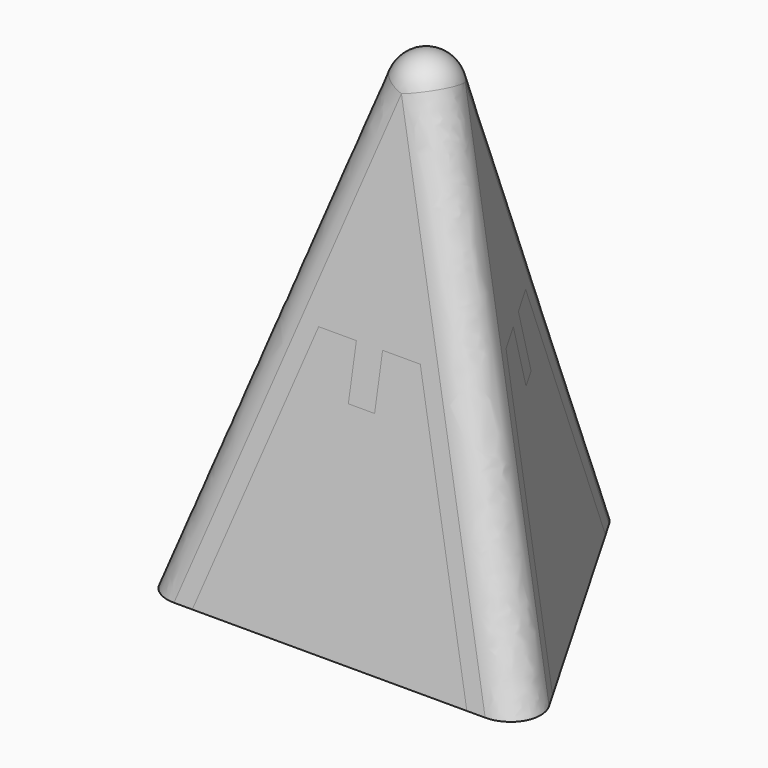
from build123d import *

# Parameters (mm, degrees)
F3_DEPTH        = 4
F5_DEPTH        = 4
F7_DEPTH        = 4
F8_DEPTH        = 2
F8_COPIES_COUNT = 3
F10_W           = 40
F10_H           = 6
F11_DEPTH       = 25
F11_DEPTH_BACK  = 25
F12_R           = 3


# Not quite as in the source:
# - an extrude whose draft closes it to a point is written as a loft to that point
# - a feature of the source that left no trace in its solid (it failed there, or was rolled back) is left out
# - a pattern or mirror of a feature is missing from the dataset's text; its kind, count and spacing are read off the source's solid


with BuildPart() as f0:
    # F13 (on Top) → F0 section 0
    with BuildSketch(Plane.XY, mode=Mode.PRIVATE) as f0_s0:
        Polygon((-21.5980762114, -12.4696551146), (21.5980762114, -12.4696551146), (0, 24.9393102292), align=None)
    loft([f0_s0.sketch, Vertex(0, 0, 64.1508142976)], ruled=True)

    # F1 (on face) → F3 (cut)
    with BuildSketch(Plane(origin=(0, -12.0156590044, 2.3356075118), x_dir=(1, 0, 0), z_dir=(0, -0.9816271834, 0.1908089954))):
        Polygon((-4.8375685578, 27.6206776349), (-14.7522947938, -2.3793223651), (0, -2.3793223651), (14.7522947938, -2.3793223651), (4.8375685578, 27.6206776349), (1.25, 27.6206776349), (1.25, 22.6206776349), (0, 22.6206776349), (-1.25, 22.6206776349), (-1.25, 27.6206776349), align=None)
    extrude(amount=-F3_DEPTH, mode=Mode.SUBTRACT)

    # F4 (on face) → F5 (cut)
    with BuildSketch(Plane(origin=(10.4058659411, 6.0078295022, 2.3356075118), x_dir=(-0.4788987638, 0.8712646086, -0.1074893292), z_dir=(0.8501140779, 0.4908135917, 0.1908089954))):
        Polygon((-7.8329752774, 26.9248658467), (-14.40304573, -3.980408308), (0.2605385928, -2.3650147058), (14.9241229157, -0.7496211036), (1.7839820104, 27.9843047215), (-1.7820133006, 27.5914617519), (-1.2345074295, 22.6215284202), (-2.4769907625, 22.4846519525), (-3.7194740954, 22.3477754847), (-4.2669799664, 27.3177088164), align=None)
    extrude(amount=-F5_DEPTH, mode=Mode.SUBTRACT)

    # F6 (on face) → F7 (cut)
    with BuildSketch(Plane(origin=(-10.4058659411, 6.0078295022, 2.3356075118), x_dir=(-0.4788987638, -0.8712646086, 0.1074893292), z_dir=(-0.8501140779, 0.4908135917, 0.1908089954))):
        Polygon((-1.7839820104, 27.9843047215), (-14.9241229157, -0.7496211036), (-0.2605385928, -2.3650147058), (14.40304573, -3.980408308), (7.8329752774, 26.9248658467), (4.2669799664, 27.3177088164), (3.7194740954, 22.3477754847), (2.4769907625, 22.4846519525), (1.2345074295, 22.6215284202), (1.7820133006, 27.5914617519), align=None)
    extrude(amount=-F7_DEPTH, mode=Mode.SUBTRACT)

    # F1 (on face) → F8 (join)
    with BuildSketch(Plane(origin=(0, -12.0156590044, 2.3356075118), x_dir=(1, 0, 0), z_dir=(0, -0.9816271834, 0.1908089954))):
        Polygon((-4.8375685578, 27.6206776349), (-14.7522947938, -2.3793223651), (0, -2.3793223651), (14.7522947938, -2.3793223651), (4.8375685578, 27.6206776349), (1.25, 27.6206776349), (1.25, 22.6206776349), (0, 22.6206776349), (-1.25, 22.6206776349), (-1.25, 27.6206776349), align=None)
    f8 = extrude(amount=-F8_DEPTH)

    # F8_copies: F8 ×3 about axis
    f8_copies_axis = Axis((0, 0, 0), (0, 0, 1))
    for i in range(1, F8_COPIES_COUNT):
        add(f8.rotate(f8_copies_axis, i * 360 / F8_COPIES_COUNT))

    # F10 (on Right) → F11 (cut, two sides)
    with BuildSketch(Plane.YZ) as f11_sk:
        with Locations((6, 2)):
            Rectangle(F10_W, F10_H)
    extrude(amount=-F11_DEPTH, mode=Mode.SUBTRACT)
    extrude(f11_sk.sketch, amount=F11_DEPTH_BACK, mode=Mode.SUBTRACT)

    # F12
    f12_edges = [f0.edges().sort_by_distance(p)[0] for p in [
        (-9.957347, -5.748877, 34.575407),
        (9.957347, -5.748877, 34.575407),
        (0, 11.497754, 34.575407),
    ]]
    fillet(f12_edges, radius=F12_R)


solid = f0.part
